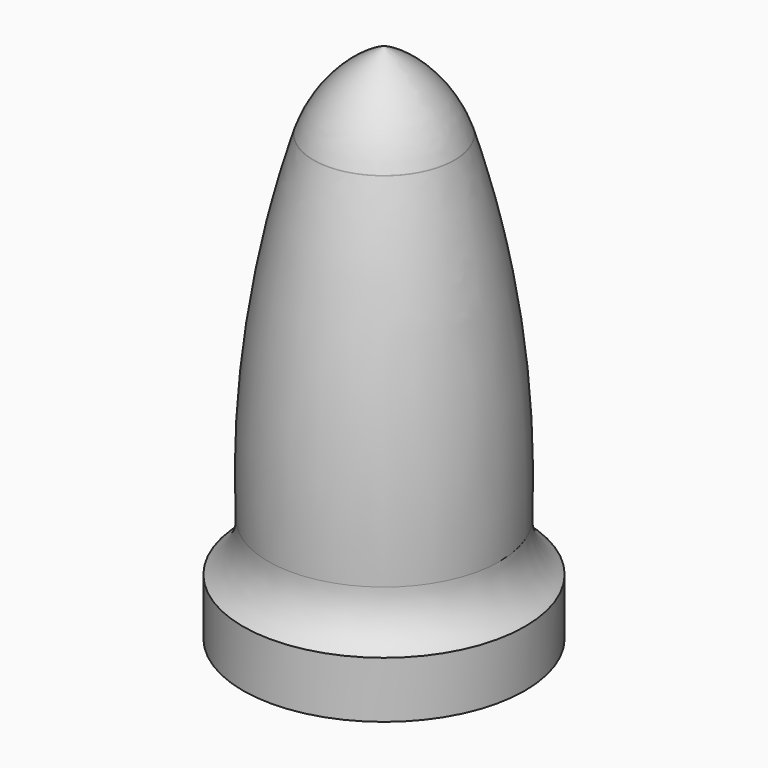
from build123d import *

# Parameters (mm, degrees)
F5_D     = 6.6
F5_DEPTH = 15.7
F5_TIP   = 1.9828400428


# Not quite as in the source:
# - a fillet or chamfer that OpenCascade refuses, or shapes differently, is made with other operations: its cross-section is extruded or revolved along the edge and cut away or added


with BuildPart() as f1:
    # F0 (on Front) → F1 (revolve)
    with BuildSketch(Plane.XZ):
        with BuildLine():
            Line((0, 39.9755910039), (0, 0))
            Line((0, 0), (12.7, 0))
            Line((12.7, 0), (12.7, 5.08))
            Line((12.7, 5.08), (10.16, 5.08))
            ThreePointArc((10.16, 5.08), (9.9566084979, 22.7135819635), (6.35, 39.9755910039))
            ThreePointArc((6.35, 39.9755910039), (3.8962255036, 44.1122905365), (0, 46.9323471189))
            Line((0, 46.9323471189), (0, 39.9755910039))
        make_face()
    revolve(axis=Axis((0, 0, 19.9877955019), (0, 0, 1)))

    # F2: fillet of radius 5.08 on 2 edges, made by hand

    # F2_s1 → F2_t2 (revolve, cut)
    with BuildSketch(Plane.XZ):
        with BuildLine():
            ThreePointArc((6.3148018826, 40.0777532467), (6.3459787539, 39.9869130594), (6.3754335423, 39.895499973))
            Line((6.3754335423, 39.895499973), (6.8606325436, 40.0467938152))
            ThreePointArc((6.8606325436, 40.0467938152), (6.847664113, 40.0870070025), (6.8350588395, 40.1273336142))
            Line((6.8350588395, 40.1273336142), (6.8306622812, 40.1407323647))
            ThreePointArc((6.8306622812, 40.1407323647), (6.8122324735, 40.1939788871), (6.793937718, 40.2472724163))
            Line((6.793937718, 40.2472724163), (6.3148018826, 40.0777532467))
        make_face()
    revolve(axis=Axis((0, 0, 39.9755910039), (0, 0, 1)), mode=Mode.SUBTRACT)

    # F3: fillet of radius 5.08 on 1 edges, made by hand

    # F3_s1 → F3_t2 (revolve)
    with BuildSketch(Plane.XZ):
        with BuildLine():
            ThreePointArc((10.4313556507, 9.5009663488), (10.9882364338, 6.9941657979), (12.7, 5.08))
            Line((12.7, 5.08), (10.16, 5.08))
            ThreePointArc((10.16, 5.08), (10.3226272558, 7.2888290382), (10.4313556507, 9.5009663488))
        make_face()
    revolve(axis=Axis((0, 0, 5.08), (0, 0, 1)))

    # F5
    with Locations(Plane(origin=(0, 0, 0), x_dir=(1, 0, 0), z_dir=(0, 0, -1))):
        with Locations((0, 0)):
            Hole(F5_D / 2, depth=F5_DEPTH)
            with Locations((0, 0, -(F5_DEPTH + F5_TIP / 2))):  # 118° drill point
                Cone(0, F5_D / 2, F5_TIP, mode=Mode.SUBTRACT)


solid = f1.part
